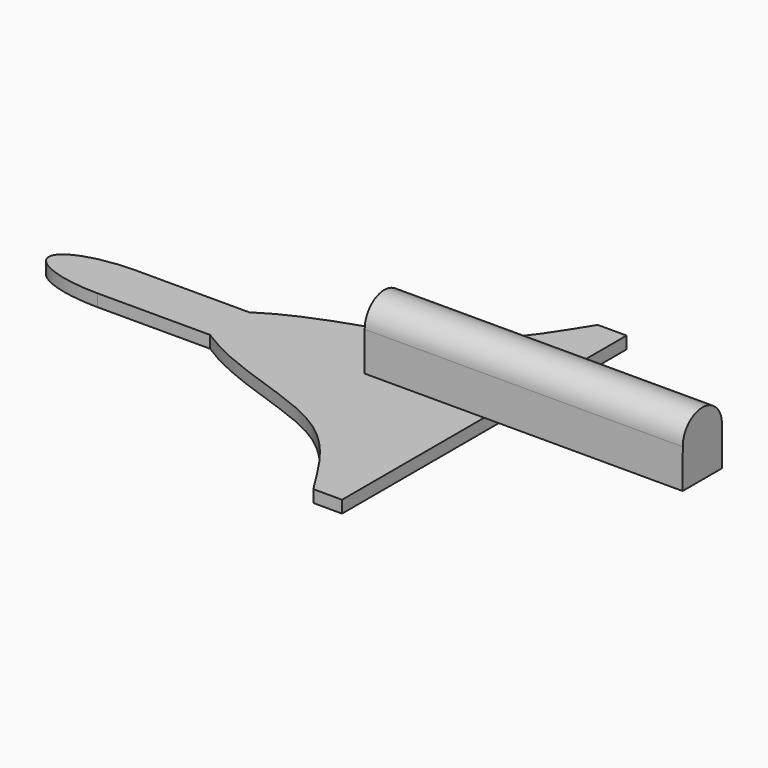
from build123d import *

# Parameters (mm, degrees)
F1_DEPTH = 5
F3_DEPTH = 130


# Not quite as in the source:
# - a feature names something its author has since deleted; it is built from what else it names


with BuildPart() as f1:
    # F0 (on Top) → F1 (new body)
    with BuildSketch(Plane.XY):
        with BuildLine():
            Line((40.8830098808, -10), (-63.2155463099, -10))
            add(Edge.make_bspline(
                [(-63.2155463099, -10), (-42.3123203218, -23.7419363111), (4.2183280181, -29.5239745011), (21.0766339926, -60.0394110264), (29.1229858994, -72.6713687181)],
                knots=[0, 0, 0, 0, 0.551730828, 1, 1, 1, 1], degree=3))
            Line((29.1229858994, -72.6713687181), (40.8830098808, -72.6713687181))
            Line((40.8830098808, -72.6713687181), (40.8830098808, -10))
        make_face()
        with BuildLine():
            Line((-63.2155463099, 10), (-109.1169901192, 10))
            add(Edge.make_bspline(
                [(-81.1169901192, 0), (-81.1169901192, 10), (-109.1169901192, 10)],
                knots=[0, 0, 0, 1.5707963268, 1.5707963268, 1.5707963268], degree=2, weights=[1, 0.7071067812, 1]))
            add(Edge.make_bspline(
                [(-109.1169901192, -10), (-81.1169901192, -10), (-81.1169901192, 0)],
                knots=[4.7123889804, 4.7123889804, 4.7123889804, 6.2831853072, 6.2831853072, 6.2831853072], degree=2, weights=[1, 0.7071067812, 1]))
            Line((-109.1169901192, -10), (-63.2155463099, -10))
            Line((-63.2155463099, -10), (40.8830098808, -10))
            Line((40.8830098808, -10), (40.8830098808, 0))
            Line((40.8830098808, 0), (40.8830098808, 10))
            Line((40.8830098808, 10), (-63.2155463099, 10))
        make_face()
        with BuildLine():
            add(Edge.make_bspline(
                [(-63.2155463099, 10), (-42.3123203218, 23.7419363111), (4.2183280181, 29.5239745011), (21.0766339926, 60.0394110264), (29.1229858994, 72.6713687181)],
                knots=[0, 0, 0, 0, 0.551730828, 1, 1, 1, 1], degree=3))
            Line((-63.2155463099, 10), (40.8830098808, 10))
            Line((40.8830098808, 10), (40.8830098808, 72.6713687181))
            Line((40.8830098808, 72.6713687181), (29.1229858994, 72.6713687181))
        make_face()
        with BuildLine():
            add(Edge.make_bspline(
                [(-81.1169901192, 0), (-81.1169901192, 10), (-109.1169901192, 10)],
                knots=[0, 0, 0, 1.5707963268, 1.5707963268, 1.5707963268], degree=2, weights=[1, 0.7071067812, 1]))
            add(Edge.make_bspline(
                [(-109.1169901192, 10), (-137.1169901192, 10), (-137.1169901192, 0)],
                knots=[1.5707963268, 1.5707963268, 1.5707963268, 3.1415926536, 3.1415926536, 3.1415926536], degree=2, weights=[1, 0.7071067812, 1]))
            Line((-137.1169901192, 0), (-81.1169901192, 0))
        make_face()
        with BuildLine():
            add(Edge.make_bspline(
                [(-109.1169901192, -10), (-81.1169901192, -10), (-81.1169901192, 0)],
                knots=[4.7123889804, 4.7123889804, 4.7123889804, 6.2831853072, 6.2831853072, 6.2831853072], degree=2, weights=[1, 0.7071067812, 1]))
            Line((-81.1169901192, 0), (-137.1169901192, 0))
            add(Edge.make_bspline(
                [(-137.1169901192, 0), (-137.1169901192, -10), (-109.1169901192, -10)],
                knots=[3.1415926536, 3.1415926536, 3.1415926536, 4.7123889804, 4.7123889804, 4.7123889804], degree=2, weights=[1, 0.7071067812, 1]))
        make_face()
    extrude(amount=F1_DEPTH)


with BuildPart() as f3:
    # F2 (on Right) → F3 (new body)
    with BuildSketch(Plane.YZ):
        with BuildLine():
            Line((9.9135860801, 11.6713725179), (10, 27.6713725179))
            ThreePointArc((10, 27.6713725179), (0.0517808517, 17.6715065817), (-9.9994637487, 27.5678122029))
            Line((-9.9994637487, 27.5678122029), (-10.0864139199, 11.6713725179))
            Line((-10.0864139199, 11.6713725179), (9.9135860801, 11.6713725179))
        make_face()
        with BuildLine():
            ThreePointArc((-9.9994637487, 27.5678122029), (0.0517808517, 17.6715065817), (10, 27.6713725179))
            ThreePointArc((10, 27.6713725179), (-0.0517808517, 37.6712384542), (-9.9994637487, 27.5678122029))
        make_face()
    extrude(amount=F3_DEPTH)


solid = Compound([f1.part, f3.part])
